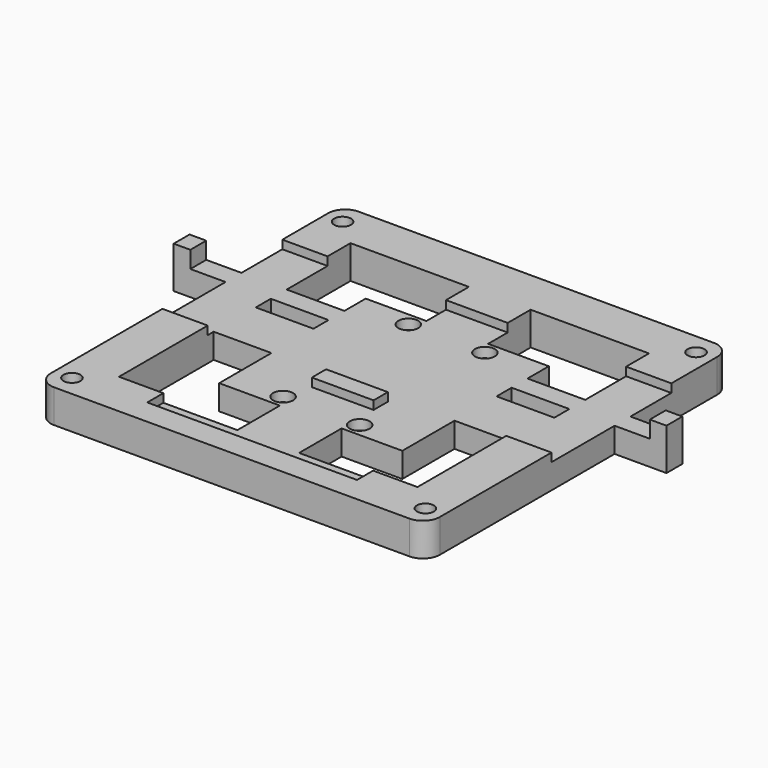
from build123d import *

# Parameters (mm, degrees)
F0_W             = 116.84
F0_H             = 114.3
F1_DEPTH         = 10.0000054
F3_R             = 5.08
F4_R             = 2.54
F5_DEPTH         = 21.59
F6_W             = 35.56
F6_H             = 35.56
F7_DEPTH         = 53.086
F7_COPIES2_COUNT = 2
F8_W             = 138
F8_H             = 45
F8_W_2           = 63
F8_H_2           = 34
F9_DEPTH         = 2.54
F10_W            = 148
F10_H            = 5.96314
F11_DEPTH        = 7.46
F12_W            = 5
F12_H            = 5.96314
F13_DEPTH        = 5.08
F14_W            = 55
F14_H            = 55
F15_DEPTH        = 7.46
F16_R            = 1.5
F17_DEPTH        = 25
F18_R            = 3
F19_DEPTH        = 3


# Not quite as in the source:
# - a pattern or mirror of a feature is missing from the dataset's text; its kind, count and spacing are read off the source's solid


with BuildPart() as f1:
    # F0 (on Top) → F1 (new body)
    with BuildSketch(Plane.XY):
        Rectangle(F0_W, F0_H)
    extrude(amount=F1_DEPTH)

    # F3
    f3_edges = [f1.edges().sort_by_distance(p)[0] for p in [
        (58.42, -57.15, 5.000003),
        (-58.42, -57.15, 5.000003),
        (58.42, 57.15, 5.000003),
        (-58.42, 57.15, 5.000003),
    ]]
    fillet(f3_edges, radius=F3_R)

    # F4 (on face) → F5 (cut)
    with BuildSketch(Plane.XY.offset(10.0000054)):
        with Locations((53.08092, -50.8)):
            Circle(F4_R)
    f5 = extrude(amount=-F5_DEPTH, mode=Mode.SUBTRACT)

    # F5_copies: F5 across plane
    add(f5.mirror(Plane(origin=(0, 0, 0), x_dir=(-0.6914141427, -0.7224586377, 0), z_dir=(-0.7224586377, 0.6914141427, 0))), mode=Mode.SUBTRACT)

    # F5_copies1: F5 across plane
    add(f5.mirror(Plane.ZX), mode=Mode.SUBTRACT)

    # F5_copies2: F5 across plane
    add(f5.mirror(Plane(origin=(0, 0, 0), x_dir=(0, 0, -1), z_dir=(-1, 0, 0))), mode=Mode.SUBTRACT)

    # F6 (on Top) → F7 (cut)
    with BuildSketch(Plane.XY):
        with Locations((27.0513010406, -25.6779607099)):
            Rectangle(F6_W, F6_H)
    f7 = extrude(amount=F7_DEPTH, mode=Mode.SUBTRACT)

    # F7_copies: F7 across plane
    add(f7.mirror(Plane(origin=(0, 0, 0), x_dir=(0, 0, -1), z_dir=(-1, 0, 0))), mode=Mode.SUBTRACT)

    # F7_copies1: F7 across plane
    add(f7.mirror(Plane(origin=(0, 3.2e-05, 0), x_dir=(1, -1e-06, 0), z_dir=(1e-06, 1, 0))), mode=Mode.SUBTRACT)

    # F7_copies2: F7 ×2 about axis
    f7_copies2_axis = Axis((0, 0, 0), (0, 0, 1))
    for i in range(1, F7_COPIES2_COUNT):
        add(f7.rotate(f7_copies2_axis, i * 360 / F7_COPIES2_COUNT), mode=Mode.SUBTRACT)

    # F8 (on face) → F9 (cut)
    with BuildSketch(Plane.XY.offset(10.0000054)):
        with Locations((0, 12.3546994664)):
            Rectangle(F8_W, F8_H)
        with Locations((0, -32.502643764)):
            Rectangle(F8_W_2, F8_H_2)
    extrude(amount=-F9_DEPTH, mode=Mode.SUBTRACT)

    # F10 (on face) → F11 (join)
    with BuildSketch(Plane.XY.offset(7.4600054)):
        with Locations((0, 16.5256112814)):
            Rectangle(F10_W, F10_H)
    extrude(amount=-F11_DEPTH)

    # F12 (on face) → F13 (join)
    with BuildSketch(Plane.XY.offset(7.4600054)):
        with Locations((71.5, 16.5256112814)):
            Rectangle(F12_W, F12_H)
        with Locations((-71.5, 16.5256112814)):
            Rectangle(F12_W, F12_H)
    extrude(amount=F13_DEPTH)

    # F14 (on face) → F15 (join)
    with BuildSketch(Plane.XY.offset(7.4600054)):
        Rectangle(F14_W, F14_H)
    extrude(amount=-F15_DEPTH)

    # F16 (on face) → F17 (cut)
    with BuildSketch(Plane.XY.offset(7.4600054)):
        with Locations((11.5, 23.5)):
            Circle(F16_R)
        with Locations((-11.5, -23.5)):
            Circle(F16_R)
        with Locations((11.5, -23.5)):
            Circle(F16_R)
        with Locations((-11.5, 23.5)):
            Circle(F16_R)
    extrude(amount=-F17_DEPTH, mode=Mode.SUBTRACT)

    # F18 (on face) → F19 (cut)
    with BuildSketch(Plane.XY.offset(7.4600054)):
        with Locations((11.5, 23.5)):
            Circle(F18_R)
        with Locations((-11.5, 23.5)):
            Circle(F18_R)
        with Locations((-11.5, -23.5)):
            Circle(F18_R)
        with Locations((11.5, -23.5)):
            Circle(F18_R)
    extrude(amount=-F19_DEPTH, mode=Mode.SUBTRACT)


solid = f1.part
